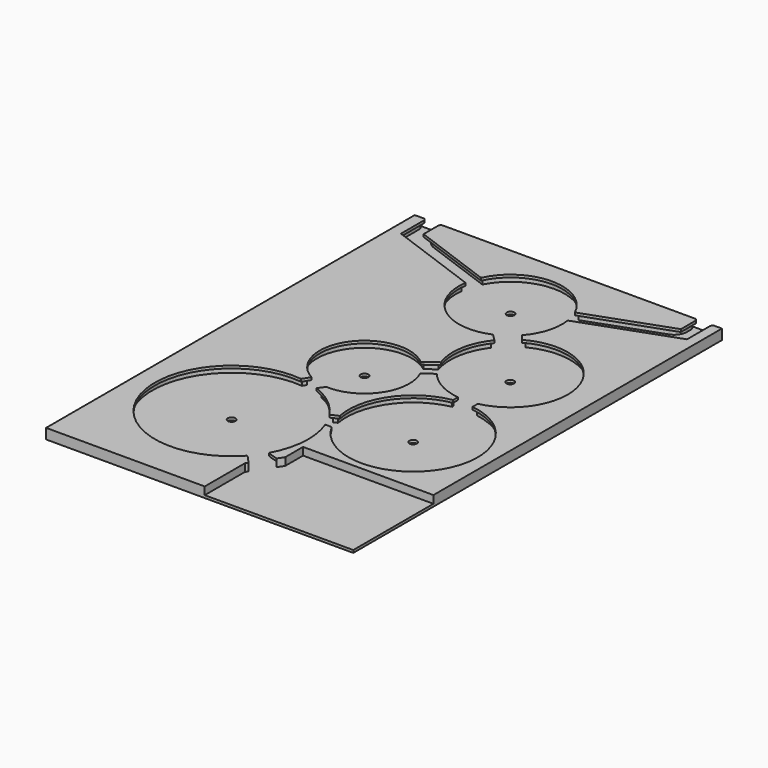
from build123d import *

# Parameters (mm, degrees)
F0_W          = 120
F0_H          = 180
F1_DEPTH      = 1
F3_DEPTH      = 2
F4_R          = 1.5
F5_DEPTH      = 1
F7_DEPTH      = 1
F8_R          = 1
F9_R          = 2
F10_T4_DEPTH  = 19.4793405237
F10_T10_DEPTH = 10.7839076458
F10_T12_DEPTH = 2
F10_T14_DEPTH = 2
F10_T16_DEPTH = 2


# Not quite as in the source:
# - a fillet or chamfer that OpenCascade refuses, or shapes differently, is made with other operations: its cross-section is extruded or revolved along the edge and cut away or added


with BuildPart() as f1:
    # F0 (on Top) → F1 (new body)
    with BuildSketch(Plane.XY):
        Rectangle(F0_W, F0_H)
    extrude(amount=F1_DEPTH)

    # F2 (on face) → F3 (join)
    with BuildSketch(Plane.XY.offset(1)):
        with BuildLine():
            ThreePointArc((5.7743163641, 19.4125560874), (4.9832762743, 30.4122392819), (9.3102960102, 40.5559898216))
            Line((9.3102960102, 40.5559898216), (7.7456061238, 42.095956144))
            ThreePointArc((7.7456061238, 42.095956144), (-12.8527116408, 44.9745444723), (-21.0559435865, 64.086947543))
            Line((-21.0559435865, 64.086947543), (-56.6113785743, 77.083993049))
            Line((-56.6113785743, 77.083993049), (-56.6113785743, 90))
            Line((-56.6113785743, 90), (-60, 90))
            Line((-60, 90), (-60, -90))
            Line((-60, -90), (1.9673409406, -90))
            Line((1.9673409406, -90), (1.9673409406, -70.4346411675))
            Line((1.9673409406, -70.4346411675), (2.616505266, -69.4407183096))
            Line((2.616505266, -69.4407183096), (-0.5101646957, -67.3985853814))
            ThreePointArc((-0.5101646957, -67.3985853814), (-51.8128586727, -56.7109367212), (-19.9826654378, -15.0812472939))
            Line((-19.9826654378, -15.0812472939), (-19.0795193014, -13.6503895026))
            ThreePointArc((-19.0795193014, -13.6503895026), (-24.4245614448, 12.5595430325), (1.9975642587, 16.731031054))
            Line((1.9975642587, 16.731031054), (5.7743163641, 19.4125560874))
        make_face()
        with BuildLine():
            ThreePointArc((3.893983022, -27.2884377194), (8.1177507192, -8.1345994764), (24.4460798679, 2.7325712784))
            Line((24.4460798679, 2.7325712784), (24.4460798679, 3.3956557663))
            ThreePointArc((24.4460798679, 3.3956557663), (16.8725336469, 5.9731034829), (10.6070882692, 10.9476419853))
            Line((10.6070882692, 10.9476419853), (7.8995626137, 9.0434923179))
            ThreePointArc((7.8995626137, 9.0434923179), (6.0327541508, -8.4723711354), (-9.6512998226, -16.4911551649))
            Line((-9.6512998226, -16.4911551649), (-10.4094366834, -17.5399380287))
            ThreePointArc((-10.4094366834, -17.5399380287), (-3.2805892037, -21.8805224353), (2.4296782432, -27.9677208929))
            Line((2.4296782432, -27.9677208929), (3.893983022, -27.2884377194))
        make_face()
        with BuildLine():
            Line((57.1415945888, 77.083993049), (21.0559435865, 64.086947543))
            ThreePointArc((21.0559435865, 64.086947543), (20.3135472344, 55.8154256572), (16.4477156209, 48.4652846663))
            Line((16.4477156209, 48.4652846663), (17.3551916053, 47.3757231641))
            ThreePointArc((17.3551916053, 47.3757231641), (50.0032635247, 34.8844107262), (33.9259108744, 3.8449484526))
            Line((33.9259108744, 3.8449484526), (33.9259108744, 2.9428404548))
            ThreePointArc((33.9259108744, 2.9428404548), (51.375757227, -37.7966835864), (7.0876050588, -36.1336939998))
            Line((7.0876050588, -36.1336939998), (6.5756302201, -36.1336939998))
            ThreePointArc((6.5756302201, -36.1336939998), (8.0704516148, -48.269522221), (4.7498989473, -60.0375614629))
            Line((4.7498989473, -60.0375614629), (7.5594950835, -61.8726028504))
            Line((7.5594950835, -61.8726028504), (9.0734828264, -59.5545656979))
            Line((9.0734828264, -59.5545656979), (9.0734828264, -50.869282335))
            Line((9.0734828264, -50.869282335), (60, -50.869282335))
            Line((60, -50.869282335), (60, 90))
            Line((60, 90), (57.1415945888, 90))
            Line((57.1415945888, 90), (57.1415945888, 77.083993049))
        make_face()
        with BuildLine():
            Line((-49.0309594103, 82.5642955171), (-18.820212287, 71.520964019))
            ThreePointArc((-18.820212287, 71.520964019), (0, 82.9866549619), (18.820212287, 71.520964019))
            Line((18.820212287, 71.520964019), (49.4814734299, 82.5642955171))
            Line((49.4814734299, 82.5642955171), (49.4814734299, 90))
            Line((49.4814734299, 90), (-49.0309594103, 90))
            Line((-49.0309594103, 90), (-49.0309594103, 82.5642955171))
        make_face()
    extrude(amount=F3_DEPTH)

    # F4 (on face) → F5 (cut, through all)
    with BuildSketch(Plane.XY.offset(1)):
        with Locations((-9.2187389006, 2.0105171313)):
            Circle(F4_R)
        with Locations((29.7579686112, -22.9492865482)):
            Circle(F4_R)
        with Locations((-22.7985265463, -45.9118092327)):
            Circle(F4_R)
        with Locations((28.0994249015, 26.5463472953)):
            Circle(F4_R)
        with Locations((0, 61.8077106774)):
            Circle(F4_R)
    extrude(amount=-F5_DEPTH, mode=Mode.SUBTRACT)

    # F6 (on face) → F7 (join)
    with BuildSketch(Plane.XY.offset(3)):
        with BuildLine():
            Line((-50.0309594103, 81.8651218962), (-18.3176540037, 70.2725405185))
            ThreePointArc((-18.3176540037, 70.2725405185), (-0.0021397414, 81.9866548485), (18.315858399, 70.2764250748))
            Line((18.315858399, 70.2764250748), (50.4814734299, 81.8615829055))
            Line((50.4814734299, 81.8615829055), (50.4814734299, 89))
            Line((50.4814734299, 89), (50.4814734299, 90))
            Line((50.4814734299, 90), (49.4814734299, 90))
            Line((49.4814734299, 90), (49.4814734299, 82.5642955171))
            Line((49.4814734299, 82.5642955171), (18.820212287, 71.520964019))
            ThreePointArc((18.820212287, 71.520964019), (0, 82.9866549619), (-18.820212287, 71.520964019))
            Line((-18.820212287, 71.520964019), (-49.0309594103, 82.5642955171))
            Line((-49.0309594103, 82.5642955171), (-49.0309594103, 90))
            Line((-49.0309594103, 90), (-50.0309594103, 90))
            Line((-50.0309594103, 90), (-50.0309594103, 89))
            Line((-50.0309594103, 89), (-50.0309594103, 81.8651218962))
        make_face()
        with BuildLine():
            ThreePointArc((-0.6656338746, -66.1026465903), (-50.8378132857, -56.4632664954), (-19.4675641491, -16.1386746862))
            Line((-19.4675641491, -16.1386746862), (-17.6842398721, -13.313347385))
            ThreePointArc((-17.6842398721, -13.313347385), (-23.6796095533, 11.8780776394), (1.9636133622, 15.4805033335))
            Line((1.9636133622, 15.4805033335), (6.9595101943, 19.0276311422))
            ThreePointArc((6.9595101943, 19.0276311422), (5.9814163542, 30.3173928166), (10.6452370769, 40.6452271729))
            Line((10.6452370769, 40.6452271729), (7.9762157892, 43.2720754273))
            ThreePointArc((7.9762157892, 43.2720754273), (-12.2991385331, 45.8101801247), (-19.9629696392, 64.752135175))
            Line((-19.9629696392, 64.752135175), (-55.6113785743, 77.78316667))
            Line((-55.6113785743, 77.78316667), (-55.6113785743, 89))
            Line((-55.6113785743, 89), (-55.6113785743, 90))
            Line((-55.6113785743, 90), (-56.6113785743, 90))
            Line((-56.6113785743, 90), (-56.6113785743, 77.083993049))
            Line((-56.6113785743, 77.083993049), (-21.0559435865, 64.086947543))
            ThreePointArc((-21.0559435865, 64.086947543), (-12.8527116408, 44.9745444723), (7.7456061238, 42.095956144))
            Line((7.7456061238, 42.095956144), (9.3102960102, 40.5559898216))
            ThreePointArc((9.3102960102, 40.5559898216), (4.9832762743, 30.4122392819), (5.7743163641, 19.4125560874))
            Line((5.7743163641, 19.4125560874), (1.9975642587, 16.731031054))
            ThreePointArc((1.9975642587, 16.731031054), (-24.4245614448, 12.5595430325), (-19.0795193014, -13.6503895026))
            Line((-19.0795193014, -13.6503895026), (-19.9826654378, -15.0812472939))
            ThreePointArc((-19.9826654378, -15.0812472939), (-51.8128586727, -56.7109367212), (-0.5101646957, -67.3985853814))
            Line((-0.5101646957, -67.3985853814), (2.616505266, -69.4407183096))
            Line((2.616505266, -69.4407183096), (0.0717437619, -66.5842526346))
            Line((0.0717437619, -66.5842526346), (-0.6656338746, -66.1026465903))
        make_face()
        with BuildLine():
            Line((56.1415945888, 89), (56.1415945888, 77.7867056607))
            Line((56.1415945888, 77.7867056607), (19.9624036934, 64.7559696929))
            ThreePointArc((19.9624036934, 64.7559696929), (19.3493201754, 56.0811409197), (15.142432038, 48.4699243388))
            Line((15.142432038, 48.4699243388), (17.1097320999, 46.1078845188))
            ThreePointArc((17.1097320999, 46.1078845188), (49.0638742633, 34.5412800266), (32.9259108744, 4.6344299996))
            Line((32.9259108744, 4.6344299996), (32.9259108744, 2.0764449012))
            ThreePointArc((32.9259108744, 2.0764449012), (50.6298931929, -37.115650126), (7.6703406758, -35.1336939998))
            Line((7.6703406758, -35.1336939998), (5.1544175427, -35.1336939998))
            ThreePointArc((5.1544175427, -35.1336939998), (7.0913247793, -47.9444525735), (3.4378931049, -60.3750431417))
            Line((3.4378931049, -60.3750431417), (4.1679904898, -60.8518942097))
            Line((4.1679904898, -60.8518942097), (7.5594950835, -61.8726028504))
            Line((7.5594950835, -61.8726028504), (4.7498989473, -60.0375614629))
            ThreePointArc((4.7498989473, -60.0375614629), (8.0704516148, -48.269522221), (6.5756302201, -36.1336939998))
            Line((6.5756302201, -36.1336939998), (7.0876050588, -36.1336939998))
            ThreePointArc((7.0876050588, -36.1336939998), (51.375757227, -37.7966835864), (33.9259108744, 2.9428404548))
            Line((33.9259108744, 2.9428404548), (33.9259108744, 3.8449484526))
            ThreePointArc((33.9259108744, 3.8449484526), (50.0032635247, 34.8844107262), (17.3551916053, 47.3757231641))
            Line((17.3551916053, 47.3757231641), (16.4477156209, 48.4652846663))
            ThreePointArc((16.4477156209, 48.4652846663), (20.3135472344, 55.8154256572), (21.0559435865, 64.086947543))
            Line((21.0559435865, 64.086947543), (57.1415945888, 77.083993049))
            Line((57.1415945888, 77.083993049), (57.1415945888, 90))
            Line((57.1415945888, 90), (56.1415945888, 90))
            Line((56.1415945888, 90), (56.1415945888, 89))
        make_face()
        with BuildLine():
            ThreePointArc((5.0170785682, -27.8698000011), (8.9577471086, -8.6778508038), (25.4460798679, 1.9049023991))
            Line((25.4460798679, 1.9049023991), (25.4460798679, 4.2666065752))
            ThreePointArc((25.4460798679, 4.2666065752), (17.3353913395, 6.8597359084), (10.7750248604, 12.2882881835))
            Line((10.7750248604, 12.2882881835), (6.6559975083, 9.3914570689))
            ThreePointArc((6.6559975083, 9.3914570689), (5.2858338993, -7.7926914407), (-10.1481498654, -15.4715229576))
            Line((-10.1481498654, -15.4715229576), (-11.9624013743, -17.9813018532))
            ThreePointArc((-11.9624013743, -17.9813018532), (-4.073652887, -22.5256176304), (2.0859408263, -29.2295391594))
            Line((2.0859408263, -29.2295391594), (5.0170785682, -27.8698000011))
        make_face()
        with BuildLine():
            ThreePointArc((10.6070882692, 10.9476419853), (16.8725336469, 5.9731034829), (24.4460798679, 3.3956557663))
            Line((24.4460798679, 3.3956557663), (24.4460798679, 2.7325712784))
            ThreePointArc((24.4460798679, 2.7325712784), (8.1177507192, -8.1345994764), (3.893983022, -27.2884377194))
            Line((3.893983022, -27.2884377194), (2.4296782432, -27.9677208929))
            ThreePointArc((2.4296782432, -27.9677208929), (-3.2805892037, -21.8805224353), (-10.4094366834, -17.5399380287))
            Line((-10.4094366834, -17.5399380287), (-9.6512998226, -16.4911551649))
            ThreePointArc((-9.6512998226, -16.4911551649), (6.0327541508, -8.4723711354), (7.8995626137, 9.0434923179))
            Line((7.8995626137, 9.0434923179), (10.6070882692, 10.9476419853))
        make_face(mode=Mode.SUBTRACT)
        with BuildLine():
            Line((49.4814734299, 90), (-49.0309594103, 90))
            Line((-49.0309594103, 90), (-49.0309594103, 82.5642955171))
            Line((-49.0309594103, 82.5642955171), (-18.820212287, 71.520964019))
            ThreePointArc((-18.820212287, 71.520964019), (0, 82.9866549619), (18.820212287, 71.520964019))
            Line((18.820212287, 71.520964019), (49.4814734299, 82.5642955171))
            Line((49.4814734299, 82.5642955171), (49.4814734299, 90))
        make_face()
        with BuildLine():
            Line((60, 90), (57.1415945888, 90))
            Line((57.1415945888, 90), (57.1415945888, 77.083993049))
            Line((57.1415945888, 77.083993049), (21.0559435865, 64.086947543))
            ThreePointArc((21.0559435865, 64.086947543), (20.3135472344, 55.8154256572), (16.4477156209, 48.4652846663))
            Line((16.4477156209, 48.4652846663), (17.3551916053, 47.3757231641))
            ThreePointArc((17.3551916053, 47.3757231641), (50.0032635247, 34.8844107262), (33.9259108744, 3.8449484526))
            Line((33.9259108744, 3.8449484526), (33.9259108744, 2.9428404548))
            ThreePointArc((33.9259108744, 2.9428404548), (51.375757227, -37.7966835864), (7.0876050588, -36.1336939998))
            Line((7.0876050588, -36.1336939998), (6.5756302201, -36.1336939998))
            ThreePointArc((6.5756302201, -36.1336939998), (8.0704516148, -48.269522221), (4.7498989473, -60.0375614629))
            Line((4.7498989473, -60.0375614629), (7.5594950835, -61.8726028504))
            Line((7.5594950835, -61.8726028504), (9.0734828264, -59.5545656979))
            Line((9.0734828264, -59.5545656979), (9.0734828264, -50.869282335))
            Line((9.0734828264, -50.869282335), (60, -50.869282335))
            Line((60, -50.869282335), (60, 90))
        make_face()
        with BuildLine():
            Line((1.9673409406, -70.4346411675), (2.616505266, -69.4407183096))
            Line((2.616505266, -69.4407183096), (-0.5101646957, -67.3985853814))
            ThreePointArc((-0.5101646957, -67.3985853814), (-51.8128586727, -56.7109367212), (-19.9826654378, -15.0812472939))
            Line((-19.9826654378, -15.0812472939), (-19.0795193014, -13.6503895026))
            ThreePointArc((-19.0795193014, -13.6503895026), (-24.4245614448, 12.5595430325), (1.9975642587, 16.731031054))
            Line((1.9975642587, 16.731031054), (5.7743163641, 19.4125560874))
            ThreePointArc((5.7743163641, 19.4125560874), (4.9832762743, 30.4122392819), (9.3102960102, 40.5559898216))
            Line((9.3102960102, 40.5559898216), (7.7456061238, 42.095956144))
            ThreePointArc((7.7456061238, 42.095956144), (-12.8527116408, 44.9745444723), (-21.0559435865, 64.086947543))
            Line((-21.0559435865, 64.086947543), (-56.6113785743, 77.083993049))
            Line((-56.6113785743, 77.083993049), (-56.6113785743, 90))
            Line((-56.6113785743, 90), (-60, 90))
            Line((-60, 90), (-60, -90))
            Line((-60, -90), (1.9673409406, -90))
            Line((1.9673409406, -90), (1.9673409406, -70.4346411675))
        make_face()
        with BuildLine():
            Line((24.4460798679, 2.7325712784), (24.4460798679, 3.3956557663))
            ThreePointArc((24.4460798679, 3.3956557663), (16.8725336469, 5.9731034829), (10.6070882692, 10.9476419853))
            Line((10.6070882692, 10.9476419853), (7.8995626137, 9.0434923179))
            ThreePointArc((7.8995626137, 9.0434923179), (6.0327541508, -8.4723711354), (-9.6512998226, -16.4911551649))
            Line((-9.6512998226, -16.4911551649), (-10.4094366834, -17.5399380287))
            ThreePointArc((-10.4094366834, -17.5399380287), (-3.2805892037, -21.8805224353), (2.4296782432, -27.9677208929))
            Line((2.4296782432, -27.9677208929), (3.893983022, -27.2884377194))
            ThreePointArc((3.893983022, -27.2884377194), (8.1177507192, -8.1345994764), (24.4460798679, 2.7325712784))
        make_face()
    extrude(amount=F7_DEPTH)

    # F8
    f8_edges = [f1.edges().sort_by_distance(p)[0] for p in [
        (-50.030959, 90, 3.5),
        (-55.611379, 90, 3.5),
        (56.141595, 90, 3.5),
        (50.481473, 90, 3.5),
    ]]
    fillet(f8_edges, radius=F8_R)

    # F9
    f9_edges = [f1.edges().sort_by_distance(p)[0] for p in [
        (-56.611379, 90, 2),
        (-49.030959, 90, 2),
        (49.481473, 90, 2),
        (57.141595, 90, 2),
    ]]
    fillet(f9_edges, radius=F9_R)

    # F10: fillet of radius 5 on 5 edges, made by hand


with BuildPart() as f10_tool2:
    # F10_s3 → F10_t4 (new body)
    with BuildSketch(Plane.XY.offset(-7.7396702619)):
        with BuildLine():
            ThreePointArc((-56.6113785743, 80.5798611538), (-55.7091284231, 77.7148225542), (-53.3280001036, 75.8837765586))
            Line((-53.3280001036, 75.8837765586), (-56.6113785743, 77.083993049))
            Line((-56.6113785743, 77.083993049), (-56.6113785743, 80.5798611538))
        make_face()
    extrude(amount=F10_T4_DEPTH)

    split(bisect_by=Plane.XY.offset(4), keep=Keep.BOTTOM)

    split(bisect_by=Plane.XY, keep=Keep.TOP)


with BuildPart() as f1_1:
    add(f1.part)

    # F10_t1: union F10_tool2
    add(f10_tool2.part)


with BuildPart() as f10_tool8:
    # F10_s9 → F10_t10 (new body)
    with BuildSketch(Plane.XY.offset(1)):
        with BuildLine():
            ThreePointArc((57.1415945888, 80.5975561073), (56.2325340038, 77.7228013869), (53.8359087076, 75.8933771496))
            Line((53.8359087076, 75.8933771496), (57.1415945888, 77.083993049))
            Line((57.1415945888, 77.083993049), (57.1415945888, 80.5975561073))
        make_face()
    extrude(amount=F10_T10_DEPTH)

    split(bisect_by=Plane.XY.offset(4), keep=Keep.BOTTOM)


with BuildPart() as f1_2:
    add(f1_1.part)

    # F10_t7: union F10_tool8
    add(f10_tool8.part)

    # F10_s13 → F10_t12 (cut)
    with BuildSketch(Plane.XY.offset(1)):
        with BuildLine():
            ThreePointArc((-49.0309594103, 86.0601636219), (-48.1287092591, 83.1951250224), (-45.7475809396, 81.3640790267))
            Line((-45.7475809396, 81.3640790267), (-49.0309594103, 82.5642955171))
            Line((-49.0309594103, 82.5642955171), (-49.0309594103, 86.0601636219))
        make_face()
    extrude(amount=F10_T12_DEPTH, mode=Mode.SUBTRACT)

    # F10_s15 → F10_t14 (cut)
    with BuildSketch(Plane.XY.offset(1)):
        with BuildLine():
            ThreePointArc((46.1757875488, 81.3736796177), (48.5724128449, 83.203103855), (49.4814734299, 86.0778585754))
            Line((49.4814734299, 86.0778585754), (49.4814734299, 82.5642955171))
            Line((49.4814734299, 82.5642955171), (46.1757875488, 81.3736796177))
        make_face()
    extrude(amount=F10_T14_DEPTH, mode=Mode.SUBTRACT)

    # F10_s17 → F10_t16 (cut)
    with BuildSketch(Plane.XY.offset(1)):
        with BuildLine():
            ThreePointArc((7.5594950835, -61.8726028504), (6.1200498347, -59.3857493388), (6.2871757091, -56.5172110429))
            ThreePointArc((6.2871757091, -56.5172110429), (5.5731904135, -58.3012523196), (4.7498989473, -60.0375614629))
            Line((4.7498989473, -60.0375614629), (7.5594950835, -61.8726028504))
        make_face()
    extrude(amount=F10_T16_DEPTH, mode=Mode.SUBTRACT)


solid = f1_2.part
